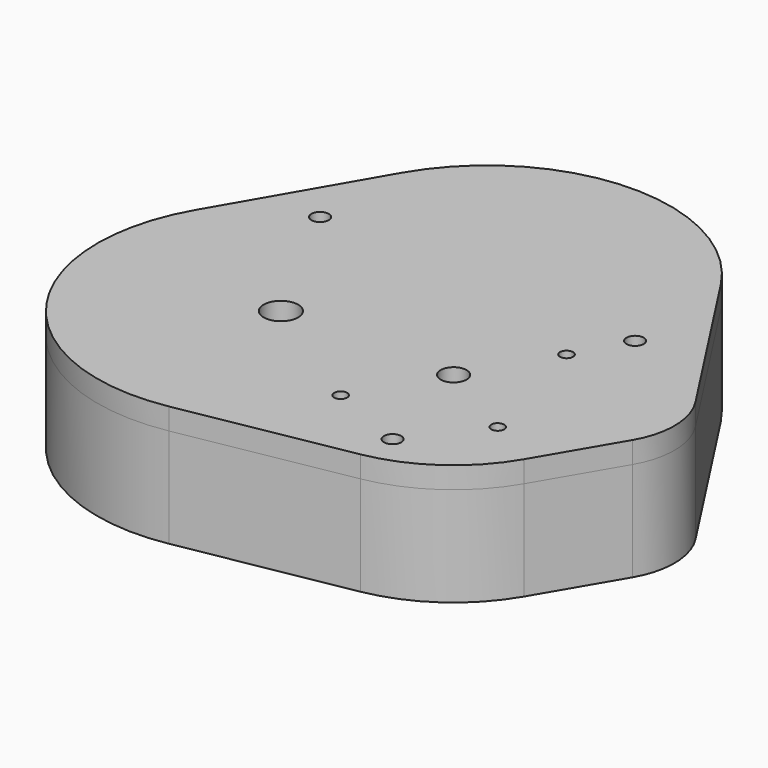
from build123d import *

# Parameters (mm, degrees)
F0_R      = 2.5
F1_DEPTH  = 8
F3_DEPTH  = 8
F5_DEPTH  = 1
F6_DEPTH  = 1
F4_R      = 4
F4_R_2    = 1.5
F4_R_3    = 3
F4_R_4    = 3.85
F4_R_5    = 10
F7_DEPTH  = 5
F8_DEPTH  = 23
F11_DEPTH = 8
F13_DEPTH = 8
F14_R     = 4
F14_R_2   = 1.5
F14_R_3   = 3
F15_DEPTH = 5
F16_DEPTH = 4
F17_R     = 1.5
F17_R_2   = 4
F17_R_3   = 3
F18_DEPTH = 4
F19_R     = 2
F20_DEPTH = 40


with BuildPart() as f1:
    # F0 (on Top) → F1 (new body)
    with BuildSketch(Plane.XY):
        with BuildLine():
            ThreePointArc((-1.95, 5.621387729), (-3.4496376621, -4.8479377059), (5.95, 0))
            ThreePointArc((5.95, 0), (4.8479377059, 3.4496376621), (1.95, 5.621387729))
            Line((1.95, 5.621387729), (-1.95, 5.621387729))
        make_face()
        Circle(F0_R, mode=Mode.SUBTRACT)
        with BuildLine():
            Line((-1.95, 5.621387729), (1.95, 5.621387729))
            ThreePointArc((1.95, 5.621387729), (0, 5.95), (-1.95, 5.621387729))
        make_face()
        with BuildLine():
            ThreePointArc((-1.95, 5.621387729), (0, 5.95), (1.95, 5.621387729))
            Line((1.95, 5.621387729), (1.95, 7.421387729))
            Line((1.95, 7.421387729), (-1.95, 7.421387729))
            Line((-1.95, 7.421387729), (-1.95, 5.621387729))
        make_face()
    extrude(amount=F1_DEPTH)

    # F2 (on face) → F3 (join, through all)
    with BuildSketch(Plane.XY.offset(8)):
        with BuildLine():
            ThreePointArc((2, 1.5), (0, 2.5), (-2, 1.5))
            Line((-2, 1.5), (2, 1.5))
        make_face()
    extrude(amount=-F3_DEPTH)

    # F5 (cut): a face of the model
    f5_faces = [f1.faces().sort_by_distance(p)[0] for p in [
        (1.7710016732, 6.521387729, 0),
    ]]
    extrude(f5_faces, amount=-F5_DEPTH, mode=Mode.SUBTRACT)

    # F6 (add): a face of the model
    f6_faces = [f1.faces().sort_by_distance(p)[0] for p in [
        (1.7710016732, 6.521387729, 8),
    ]]
    extrude(f6_faces, amount=F6_DEPTH)


with BuildPart() as f7:
    # F4 (on Top) → F7 (new body)
    with BuildSketch(Plane.XY):
        with BuildLine():
            Line((-53.3419780457, 53.8910161514), (-73.3419780457, 19.25))
            ThreePointArc((-73.3419780457, 19.25), (-71.4998043396, -22.1362220482), (-33.1857985837, -37.8921714746))
            Line((-33.1857985837, -37.8921714746), (5.5611512307, -30.9242540914))
            ThreePointArc((5.5611512307, -30.9242540914), (17.9863984999, -25.7628679134), (27.1135303231, -15.8774169038))
            Line((27.1135303231, -15.8774169038), (37.769539487, 2.3196254325))
            ThreePointArc((37.769539487, 2.3196254325), (39.6643163027, 9.6359455026), (37.4360823271, 16.8576968067))
            Line((37.4360823271, 16.8576968067), (12.2958688092, 55.5987559594))
            ThreePointArc((12.2958688092, 55.5987559594), (-21.0013390768, 73.127992131), (-53.3419780457, 53.8910161514))
        make_face()
        with Locations((-40, 0)):
            Circle(F4_R, mode=Mode.SUBTRACT)
        with Locations((-10.9601551084, -18.9835455066)):
            Circle(F4_R_2, mode=Mode.SUBTRACT)
        Circle(F4_R_3, mode=Mode.SUBTRACT)
        with Locations((18.9835455066, -10.9601551084)):
            Circle(F4_R_2, mode=Mode.SUBTRACT)
        with Locations((25.8179580932, 9.3183540446)):
            Circle(F4_R_4, mode=Mode.SUBTRACT)
        with Locations((-20, 34.6410161514)):
            Circle(F4_R_5, mode=Mode.SUBTRACT)
        with Locations((10.9601551084, 18.9835455066)):
            Circle(F4_R_2, mode=Mode.SUBTRACT)
        with Locations((-10.9601551084, -18.9835455066)):
            Circle(F4_R_2)
        Circle(F4_R_3)
        with Locations((18.9835455066, -10.9601551084)):
            Circle(F4_R_2)
        with Locations((10.9601551084, 18.9835455066)):
            Circle(F4_R_2)
    extrude(amount=F7_DEPTH)

    # F4 (on Top) → F8 (join)
    with BuildSketch(Plane.XY):
        with BuildLine():
            Line((-56.8060796608, 55.8910161514), (-76.8060796608, 21.25))
            ThreePointArc((-76.8060796608, 21.25), (-74.7725112839, -24.436089274), (-32.4778296053, -41.8290204589))
            Line((-32.4778296053, -41.8290204589), (6.269120209, -34.8611030758))
            ThreePointArc((6.269120209, -34.8611030758), (20.2761783749, -29.0426404854), (30.5652505813, -17.8987103658))
            Line((30.5652505813, -17.8987103658), (41.2212597451, 0.2983319705))
            ThreePointArc((41.2212597451, 0.2983319705), (43.663264522, 9.7276686673), (40.7914972683, 19.0351243193))
            Line((40.7914972683, 19.0351243193), (15.6512837504, 57.776183472))
            ThreePointArc((15.6512837504, 57.776183472), (-21.1053743055, 77.126638986), (-56.8060796608, 55.8910161514))
        make_face()
        with BuildLine():
            ThreePointArc((-33.1857985837, -37.8921714746), (-71.4998043396, -22.1362220482), (-73.3419780457, 19.25))
            Line((-73.3419780457, 19.25), (-53.3419780457, 53.8910161514))
            ThreePointArc((-53.3419780457, 53.8910161514), (-21.0013390768, 73.127992131), (12.2958688092, 55.5987559594))
            Line((12.2958688092, 55.5987559594), (37.4360823271, 16.8576968067))
            ThreePointArc((37.4360823271, 16.8576968067), (39.6643163027, 9.6359455026), (37.769539487, 2.3196254325))
            Line((37.769539487, 2.3196254325), (27.1135303231, -15.8774169038))
            ThreePointArc((27.1135303231, -15.8774169038), (17.9863984999, -25.7628679134), (5.5611512307, -30.9242540914))
            Line((5.5611512307, -30.9242540914), (-33.1857985837, -37.8921714746))
        make_face(mode=Mode.SUBTRACT)
    extrude(amount=F8_DEPTH)


with BuildPart() as f11:
    # F10 (on offset) → F11 (new body)
    with BuildSketch(Plane.XY.offset(6)):
        with BuildLine():
            ThreePointArc((-30.9592505938, 6.1779729827), (-2.737426946, 9.4963632097), (10.5, 34.6410161514))
            ThreePointArc((10.5, 34.6410161514), (-33.1446216898, 62.1631694216), (-39.1700931562, 10.9185051463))
            ThreePointArc((-39.1700931562, 10.9185051463), (-34.525, 9.4829781714), (-30.9592505938, 6.1779729827))
        make_face()
        with BuildLine():
            ThreePointArc((-30.9592505938, 6.1779729827), (-34.525, 9.4829781714), (-39.1700931562, 10.9185051463))
            ThreePointArc((-39.1700931562, 10.9185051463), (-35.25, 8.227241336), (-30.9592505938, 6.1779729827))
        make_face()
        with BuildLine():
            ThreePointArc((-30.9592505938, 6.1779729827), (-35.25, 8.227241336), (-39.1700931562, 10.9185051463))
            ThreePointArc((-39.1700931562, 10.9185051463), (-48.0308772852, -7.4436221042), (-29.05, 0))
            ThreePointArc((-29.05, 0), (-29.538195519, 3.2331326916), (-30.9592505938, 6.1779729827))
        make_face()
    extrude(amount=F11_DEPTH)

    # F12 (on face) → F13 (join)
    with BuildSketch(Plane.XY.offset(14)):
        with BuildLine():
            ThreePointArc((-9.87065625, -4.7405321636), (-9.5928052562, -2.3775003286), (-9.5, 0))
            ThreePointArc((-9.5, 0), (-9.5928052562, 2.3775003286), (-9.87065625, 4.7405321636))
            ThreePointArc((-9.87065625, 4.7405321636), (-10.95, 0), (-9.87065625, -4.7405321636))
        make_face()
        with BuildLine():
            ThreePointArc((-9.87065625, 4.7405321636), (-9.5928052562, 2.3775003286), (-9.5, 0))
            ThreePointArc((-9.5, 0), (-9.5928052562, -2.3775003286), (-9.87065625, -4.7405321636))
            ThreePointArc((-9.87065625, -4.7405321636), (2.4309271958, -10.6767547958), (10.95, 0))
            ThreePointArc((10.95, 0), (7.4436221042, 8.0308772852), (-0.8299068438, 10.9185051463))
            ThreePointArc((-0.8299068438, 10.9185051463), (-4.75, 8.227241336), (-9.0407494062, 6.1779729827))
            ThreePointArc((-9.0407494062, 6.1779729827), (-9.4829781714, 5.475), (-9.87065625, 4.7405321636))
        make_face()
        with BuildLine():
            ThreePointArc((-9.87065625, -4.7405321636), (-10.95, 0), (-9.87065625, 4.7405321636))
            ThreePointArc((-9.87065625, 4.7405321636), (-9.9595439395, 5.2745615624), (-10.0578962995, 5.806929136))
            ThreePointArc((-10.0578962995, 5.806929136), (-20.5413550912, 4.1458208796), (-30.9592505938, 6.1779729827))
            ThreePointArc((-30.9592505938, 6.1779729827), (-45.475, -9.4829781714), (-39.1700931562, 10.9185051463))
            ThreePointArc((-39.1700931562, 10.9185051463), (-46.1389362532, 18.9245912541), (-49.9421037005, 28.8340870154))
            ThreePointArc((-49.9421037005, 28.8340870154), (-59.5881323372, -23.3785173085), (-9.87065625, -4.7405321636))
        make_face()
        with BuildLine():
            ThreePointArc((-30.9592505938, 6.1779729827), (-20.5413550912, 4.1458208796), (-10.0578962995, 5.806929136))
            ThreePointArc((-10.0578962995, 5.806929136), (-24.75, 26.4137748154), (-49.9421037005, 28.8340870154))
            ThreePointArc((-49.9421037005, 28.8340870154), (-46.1389362532, 18.9245912541), (-39.1700931562, 10.9185051463))
            ThreePointArc((-39.1700931562, 10.9185051463), (-45.475, -9.4829781714), (-30.9592505938, 6.1779729827))
        make_face()
        with BuildLine():
            ThreePointArc((-0.8299068438, 10.9185051463), (-5.475, 9.4829781714), (-9.0407494062, 6.1779729827))
            ThreePointArc((-9.0407494062, 6.1779729827), (-4.75, 8.227241336), (-0.8299068438, 10.9185051463))
        make_face()
    extrude(amount=F13_DEPTH)


with BuildPart() as f15:
    # F14 (on face) → F15 (new body)
    with BuildSketch(Plane.XY.offset(23)):
        with BuildLine():
            ThreePointArc((6.269120209, -34.8611030758), (20.2761783749, -29.0426404854), (30.5652505813, -17.8987103658))
            Line((30.5652505813, -17.8987103658), (41.2212597451, 0.2983319705))
            ThreePointArc((41.2212597451, 0.2983319705), (43.663264522, 9.7276686673), (40.7914972683, 19.0351243193))
            Line((40.7914972683, 19.0351243193), (15.6512837504, 57.776183472))
            ThreePointArc((15.6512837504, 57.776183472), (-21.1053743055, 77.126638986), (-56.8060796608, 55.8910161514))
            Line((-56.8060796608, 55.8910161514), (-76.8060796608, 21.25))
            ThreePointArc((-76.8060796608, 21.25), (-74.7725112839, -24.436089274), (-32.4778296053, -41.8290204589))
            Line((-32.4778296053, -41.8290204589), (6.269120209, -34.8611030758))
        make_face()
        with BuildLine():
            ThreePointArc((27.1135303231, -15.8774169038), (17.9863984999, -25.7628679134), (5.5611512307, -30.9242540914))
            Line((5.5611512307, -30.9242540914), (-33.1857985837, -37.8921714746))
            ThreePointArc((-33.1857985837, -37.8921714746), (-71.4998043396, -22.1362220482), (-73.3419780457, 19.25))
            Line((-73.3419780457, 19.25), (-53.3419780457, 53.8910161514))
            ThreePointArc((-53.3419780457, 53.8910161514), (-21.0013390768, 73.127992131), (12.2958688092, 55.5987559594))
            Line((12.2958688092, 55.5987559594), (37.4360823271, 16.8576968067))
            ThreePointArc((37.4360823271, 16.8576968067), (39.6643163027, 9.6359455026), (37.769539487, 2.3196254325))
            Line((37.769539487, 2.3196254325), (27.1135303231, -15.8774169038))
        make_face(mode=Mode.SUBTRACT)
        with BuildLine():
            Line((-33.1857985837, -37.8921714746), (5.5611512307, -30.9242540914))
            ThreePointArc((5.5611512307, -30.9242540914), (17.9863984999, -25.7628679134), (27.1135303231, -15.8774169038))
            Line((27.1135303231, -15.8774169038), (37.769539487, 2.3196254325))
            ThreePointArc((37.769539487, 2.3196254325), (39.6643163027, 9.6359455026), (37.4360823271, 16.8576968067))
            Line((37.4360823271, 16.8576968067), (12.2958688092, 55.5987559594))
            ThreePointArc((12.2958688092, 55.5987559594), (-21.0013390768, 73.127992131), (-53.3419780457, 53.8910161514))
            Line((-53.3419780457, 53.8910161514), (-73.3419780457, 19.25))
            ThreePointArc((-73.3419780457, 19.25), (-71.4998043396, -22.1362220482), (-33.1857985837, -37.8921714746))
        make_face()
        with Locations((-40, 0)):
            Circle(F14_R, mode=Mode.SUBTRACT)
        with Locations((-10.9601551084, -18.9835455066)):
            Circle(F14_R_2, mode=Mode.SUBTRACT)
        Circle(F14_R_3, mode=Mode.SUBTRACT)
        with Locations((18.9835455066, -10.9601551084)):
            Circle(F14_R_2, mode=Mode.SUBTRACT)
        with Locations((10.9601551084, 18.9835455066)):
            Circle(F14_R_2, mode=Mode.SUBTRACT)
    extrude(amount=F15_DEPTH)

    # F14 (on face) → F16 (join)
    with BuildSketch(Plane.XY.offset(23)):
        with BuildLine():
            Line((-33.1857985837, -37.8921714746), (5.5611512307, -30.9242540914))
            ThreePointArc((5.5611512307, -30.9242540914), (17.9863984999, -25.7628679134), (27.1135303231, -15.8774169038))
            Line((27.1135303231, -15.8774169038), (37.769539487, 2.3196254325))
            ThreePointArc((37.769539487, 2.3196254325), (39.6643163027, 9.6359455026), (37.4360823271, 16.8576968067))
            Line((37.4360823271, 16.8576968067), (12.2958688092, 55.5987559594))
            ThreePointArc((12.2958688092, 55.5987559594), (-21.0013390768, 73.127992131), (-53.3419780457, 53.8910161514))
            Line((-53.3419780457, 53.8910161514), (-73.3419780457, 19.25))
            ThreePointArc((-73.3419780457, 19.25), (-71.4998043396, -22.1362220482), (-33.1857985837, -37.8921714746))
        make_face()
        with Locations((-40, 0)):
            Circle(F14_R, mode=Mode.SUBTRACT)
        with Locations((-10.9601551084, -18.9835455066)):
            Circle(F14_R_2, mode=Mode.SUBTRACT)
        Circle(F14_R_3, mode=Mode.SUBTRACT)
        with Locations((18.9835455066, -10.9601551084)):
            Circle(F14_R_2, mode=Mode.SUBTRACT)
        with Locations((10.9601551084, 18.9835455066)):
            Circle(F14_R_2, mode=Mode.SUBTRACT)
    extrude(amount=-F16_DEPTH)

    # F17 (on face) → F18 (cut)
    with BuildSketch(Plane(origin=(0, 0, 19), x_dir=(1, 0, 0), z_dir=(0, 0, -1))):
        with BuildLine():
            Line((8.9404538679, -53.4213284469), (34.0806673859, -14.6802692942))
            ThreePointArc((34.0806673859, -14.6802692942), (35.6653680833, -9.5442223378), (34.3178192289, -4.3409188945))
            Line((34.3178192289, -4.3409188945), (23.661810065, 13.8561234418))
            ThreePointArc((23.661810065, 13.8561234418), (15.696618625, 22.4830953413), (4.8531822524, 26.987405107))
            Line((4.8531822524, 26.987405107), (-33.893767562, 33.9553224902))
            ThreePointArc((-33.893767562, 33.9553224902), (-68.2270973952, 19.8363548224), (-69.8778764306, -17.25))
            Line((-69.8778764306, -17.25), (-49.8778764306, -51.8910161514))
            ThreePointArc((-49.8778764306, -51.8910161514), (-20.897303848, -69.1293452759), (8.9404538679, -53.4213284469))
        make_face()
        with Locations((10.9601551084, -18.9835455066)):
            Circle(F17_R, mode=Mode.SUBTRACT)
        with Locations((-40, 0)):
            Circle(F17_R_2, mode=Mode.SUBTRACT)
        Circle(F17_R_3, mode=Mode.SUBTRACT)
        with Locations((-10.9601551084, 18.9835455066)):
            Circle(F17_R, mode=Mode.SUBTRACT)
        with Locations((18.9835455066, 10.9601551084)):
            Circle(F17_R, mode=Mode.SUBTRACT)
    extrude(amount=-F18_DEPTH, mode=Mode.SUBTRACT)


with BuildPart() as f20_tool:
    # F19 (on face) → F20 (new body)
    with BuildSketch(Plane.XY.offset(28)):
        with Locations((-57.4715762198, 33.1812300013)):
            Circle(F19_R)
        with Locations((17.3124925328, 30.8956321939)):
            Circle(F19_R)
        with Locations((7.1175237403, -26.5629602229)):
            Circle(F19_R)
    extrude(amount=-F20_DEPTH)


with BuildPart() as f7_1:
    add(f7.part)

    # F20: cut by f20_tool
    add(f20_tool.part, mode=Mode.SUBTRACT)


with BuildPart() as f15_1:
    add(f15.part)

    # F20: cut by f20_tool
    add(f20_tool.part, mode=Mode.SUBTRACT)


solid = Compound([f1.part, f11.part, f7_1.part, f15_1.part])
